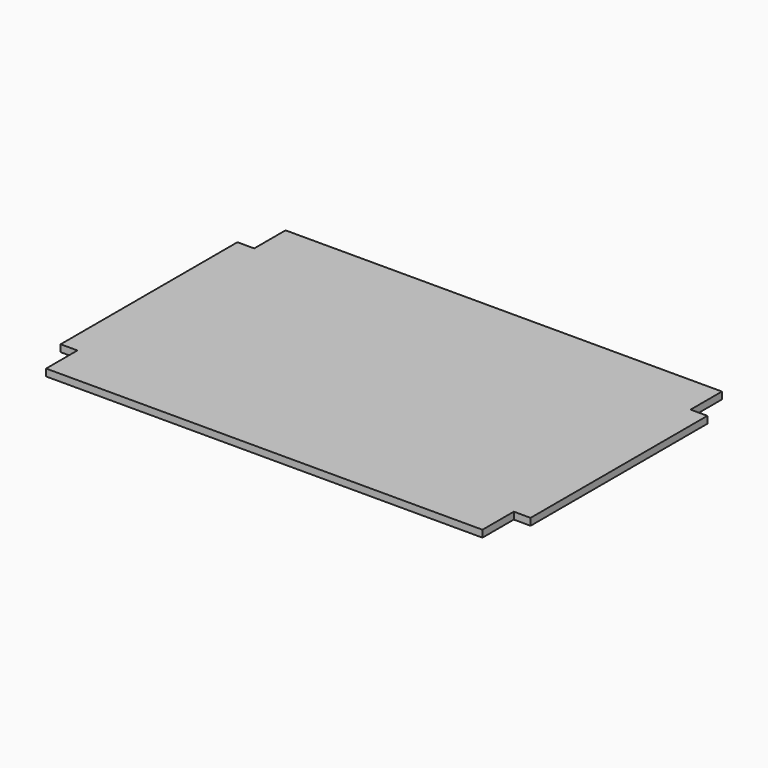
from build123d import *

# Parameters (mm, degrees)
F0_W     = 1066.8
F0_H     = 679.45
F1_DEPTH = 15.875
F2_W     = 38.1
F2_H     = 88.9
F3_DEPTH = 25.4


# Not quite as in the source:
# - a length typed as a fraction of an inch, garbled in the dataset ("3 / 203.2 mm" for 3/8 in), is restored


with BuildPart() as f1:
    # F0 (on Top) → F1 (new body)
    with BuildSketch(Plane.XY):
        with Locations((533.4, 339.725)):
            Rectangle(F0_W, F0_H)
    extrude(amount=F1_DEPTH)

    # F2 (on face) → F3 (cut)
    with BuildSketch(Plane.XY.offset(15.875)):
        with Locations((19.05, 44.45)):
            Rectangle(F2_W, F2_H)
        with Locations((19.05, 635)):
            Rectangle(F2_W, F2_H)
        with Locations((1047.75, 635)):
            Rectangle(F2_W, F2_H)
        with Locations((1047.75, 44.45)):
            Rectangle(F2_W, F2_H)
    extrude(amount=-F3_DEPTH, mode=Mode.SUBTRACT)


solid = f1.part
